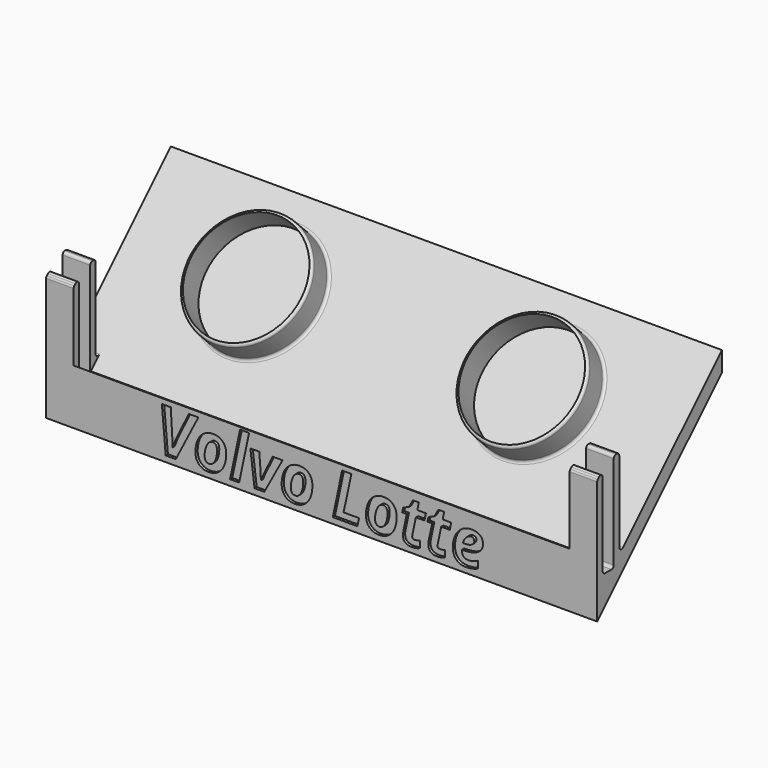
from build123d import *

# Parameters (mm, degrees)
F0_W          = 200
F0_H          = 50
F1_DEPTH      = 5
F3_DEPTH      = 200
F5_DEPTH      = 200
F7_W          = 180
F7_H          = 7.0710678119
F6_W          = 180
F6_H          = 25
F8_DEPTH      = 9
F9_DEPTH      = 5
F10_W         = 5
F10_H         = 40
F11_DEPTH     = 200
F12_R         = 21
F12_R_2       = 20
F13_DEPTH     = 10
F14_R         = 0.99999
F15_TEXT_SIZE = 22.4331824157
F16_DEPTH     = 1


# Not quite as in the source:
# - a fillet or chamfer is up to 0.001 mm smaller than in the source, because OpenCascade refuses the exact size
# - Text() gives the source's letters only with a copy of the font that has no kerning and outlines rounded to 1/6400 em; it was checked with that copy


with BuildPart() as f1:
    # F0 (on Front) → F1 (new body)
    with BuildSketch(Plane.XZ):
        Rectangle(F0_W, F0_H)
    extrude(amount=F1_DEPTH)

    # F2 (on face) → F3 (cut)
    with BuildSketch(Plane.YZ.offset(100)):
        Polygon((-5, 20), (0, 25), (-5, 25), align=None)
        Polygon((0, -25), (0, -20), (-5, -25), align=None)
    extrude(amount=-F3_DEPTH, mode=Mode.SUBTRACT)

    # F4 (on face) → F5 (join)
    with BuildSketch(Plane.YZ.offset(100)):
        Polygon((0, -12.819), (0, -20), (51.5685424949, 31.5685424949), (51.5685424949, 38.7495424949), align=None)
    extrude(amount=-F5_DEPTH)

    # F7 (on face) + F6 (on face) → F8 (cut)
    with BuildSketch(Plane(origin=(0, -12.5, 12.5), x_dir=(1, 0, 0), z_dir=(0, -0.7071067812, 0.7071067812))):
        with Locations((0, 14.1421356237)):
            Rectangle(F7_W, F7_H)
    with BuildSketch(Plane.XZ.offset(5)):
        with Locations((0, 7.5)):
            Rectangle(F6_W, F6_H)
    extrude(amount=-F8_DEPTH, dir=(0, -0.7071067812, 0.7071067812), mode=Mode.SUBTRACT)

    # F9 (add): a face of the model
    f9_faces = [f1.faces().sort_by_distance(p)[0] for p in [
        (0, 0, -10.7835571302),
    ]]
    extrude(f9_faces, amount=F9_DEPTH)

    # F10 (on face) → F11 (cut)
    with BuildSketch(Plane(origin=(-100, 0, 0), x_dir=(0, -1, 0), z_dir=(-1, 0, 0))):
        with Locations((0, 9)):
            Rectangle(F10_W, F10_H)
    extrude(amount=-F11_DEPTH, mode=Mode.SUBTRACT)

    # F12 (on face) → F13 (join)
    with BuildSketch(Plane(origin=(0, 6.4095, -6.4095), x_dir=(1, 0, 0), z_dir=(0, -0.7071067812, 0.7071067812))):
        with Locations((-50, 33.8645303601)):
            Circle(F12_R)
        with Locations((-50, 33.8645303601)):
            Circle(F12_R_2, mode=Mode.SUBTRACT)
        with Locations((50, 33.8645303601)):
            Circle(F12_R)
        with Locations((50, 33.8645303601)):
            Circle(F12_R_2, mode=Mode.SUBTRACT)
    extrude(amount=F13_DEPTH)

    # F14 (radius 1 in the source; OpenCascade refuses exactly that, so slightly less here)
    f14_edges = [f1.edges().sort_by_distance(p)[0] for p in [
        (-71, 23.284271, 24.607407),
        (29, 23.284271, 24.607407),
        (95, 5, -7.819),
        (-95, 5, -7.819),
        (0, -2.5, -11),
        (0, 2.5, -11),
        (95, 2.5, 25),
        (-95, 2.5, 25),
        (-95, -2.5, 22.5),
        (95, -2.5, 22.5),
        (-95, -5, 20),
        (-95, 5, 25),
        (95, 5, 25),
        (95, -5, 20),
        (-71, 30.355339, 17.536339),
        (29, 30.355339, 17.536339),
    ]]
    fillet(f14_edges, radius=F14_R)

    # F15 (on face) → F16 (cut)
    with BuildSketch(Plane.XZ.offset(5)):
        with Locations((-60, -22.8557434396)):
            Text('Volvo Lotte', F15_TEXT_SIZE, font='Open Sans', font_style=FontStyle.BOLDITALIC, text_align=(TextAlign.LEFT, TextAlign.BOTTOM))
    extrude(amount=-F16_DEPTH, mode=Mode.SUBTRACT)


solid = f1.part
